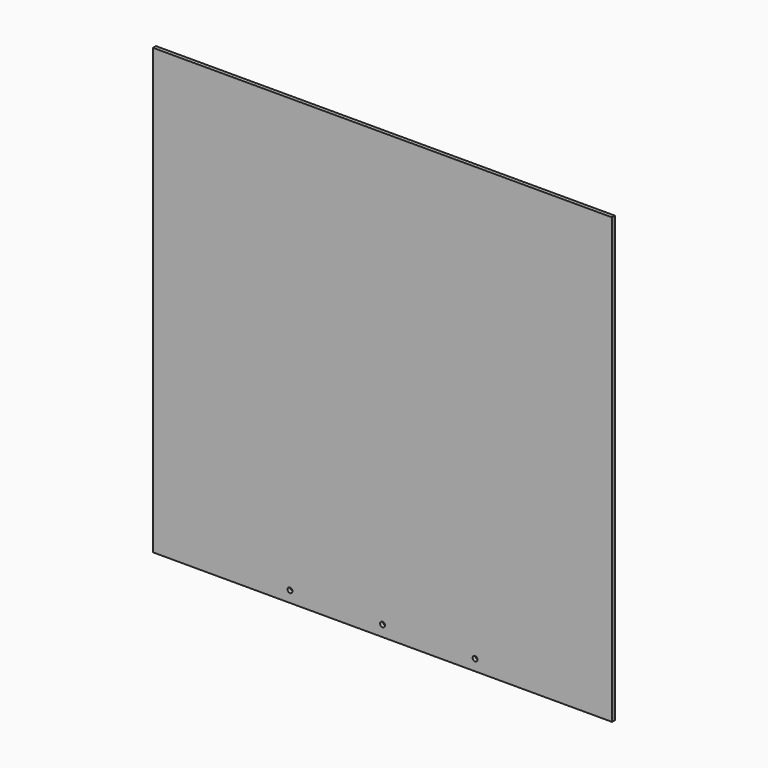
from build123d import *

# Parameters (mm, degrees)
F0_W     = 620
F0_H     = 600
F1_DEPTH = 5
F3_D     = 6.6


# Not quite as in the source:
# - a feature names something its author has since deleted; it is built from what else it names


with BuildPart() as f1:
    # F0 (on Front) → F1 (new body)
    with BuildSketch(Plane.XZ):
        Rectangle(F0_W, F0_H)
    extrude(amount=F1_DEPTH)

    # F3 (through all)
    with Locations(Plane.XZ.offset(5)):
        with Locations((-125, -285), (125, -285), (0, -285)):
            Hole(F3_D / 2)


solid = f1.part
